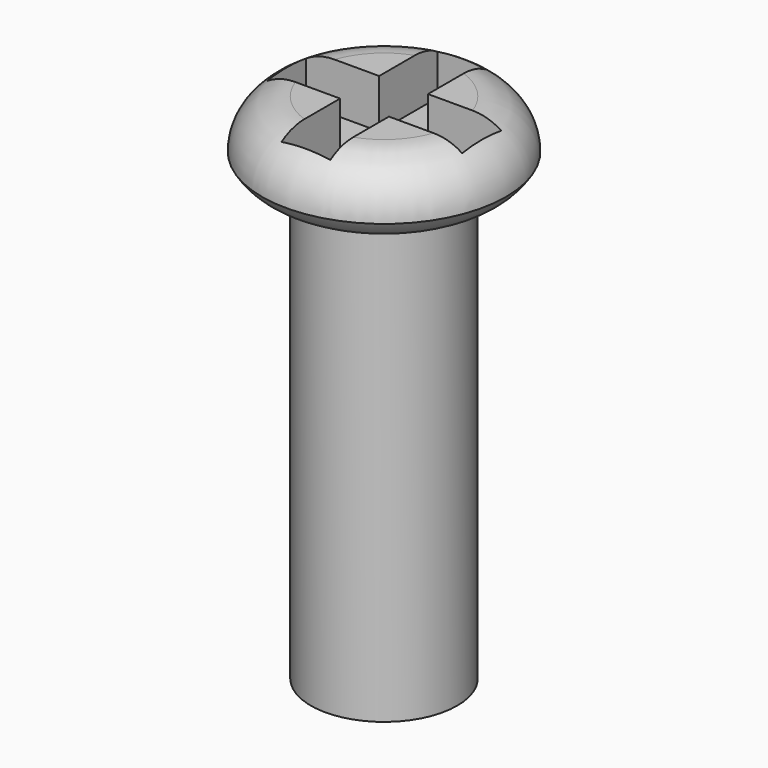
from build123d import *

# Parameters (mm, degrees)
F0_R     = 1.5
F1_DEPTH = 9
F2_R     = 2.5
F3_DEPTH = 1.5
F4_W     = 1
F4_H     = 1.5
F4_H_2   = 1
F4_W_2   = 1.5
F5_DEPTH = 1


# Not quite as in the source:
# - a fillet or chamfer that OpenCascade refuses, or shapes differently, is made with other operations: its cross-section is extruded or revolved along the edge and cut away or added


with BuildPart() as f1:
    # F0 (on Top) → F1 (new body)
    with BuildSketch(Plane.XY):
        Circle(F0_R)
    extrude(amount=F1_DEPTH)

    # F2 (on face) → F3 (join)
    with BuildSketch(Plane.XY.offset(9)):
        Circle(F2_R)
    extrude(amount=F3_DEPTH)

    # F4 (on face) → F5 (cut)
    with BuildSketch(Plane.XY.offset(10.5)):
        with Locations((0, 1.25)):
            Rectangle(F4_W, F4_H)
        Rectangle(F4_W, F4_H_2)
        with Locations((-1.25, 0)):
            Rectangle(F4_W_2, F4_H_2)
        with Locations((1.25, 0)):
            Rectangle(F4_W_2, F4_H_2)
        with Locations((0, -1.25)):
            Rectangle(F4_W, F4_H)
    extrude(amount=-F5_DEPTH, mode=Mode.SUBTRACT)

    # F6: fillet of radius 1 on 1 edges, made by hand

    # F6_s1 → F6_t2 (revolve, cut)
    with BuildSketch(Plane.XZ):
        with BuildLine():
            ThreePointArc((2.5, 9.5), (2.2071067812, 10.2071067812), (1.5, 10.5))
            Line((1.5, 10.5), (2.5, 10.5))
            Line((2.5, 10.5), (2.5, 9.5))
        make_face()
    revolve(axis=Axis((0, 0, 10.5), (0, 0, 1)), mode=Mode.SUBTRACT)

    # F7: fillet of radius 1 on 1 edges, made by hand

    # F7_s1 → F7_t2 (revolve, cut)
    with BuildSketch(Plane.XZ):
        with BuildLine():
            ThreePointArc((2.5, 9.5), (2.1339745962, 9.1339745962), (1.6339745962, 9))
            Line((1.6339745962, 9), (2.5, 9))
            Line((2.5, 9), (2.5, 9.5))
        make_face()
    revolve(axis=Axis((0, 0, 9), (0, 0, 1)), mode=Mode.SUBTRACT)


solid = f1.part
